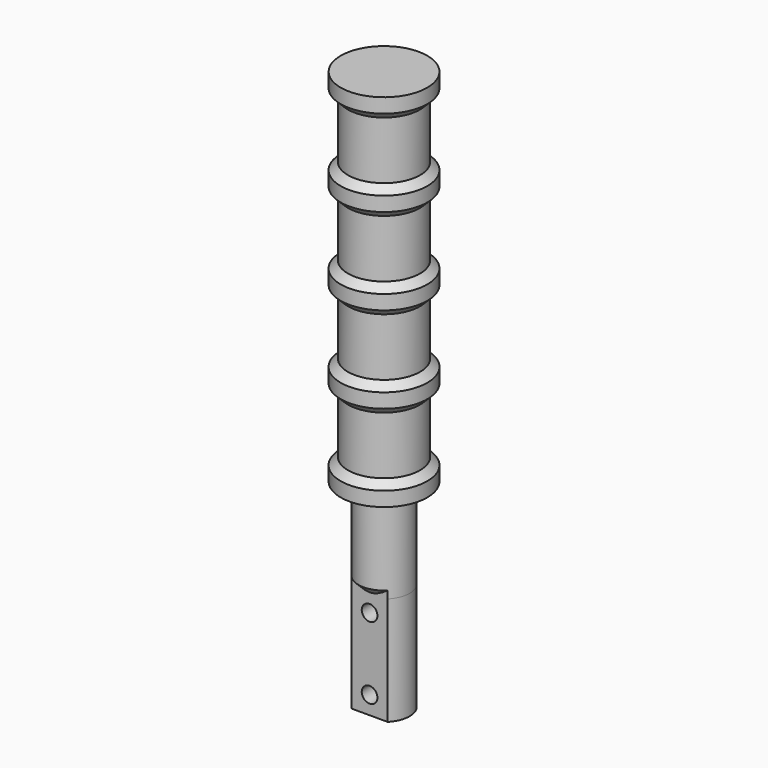
from build123d import *

# Parameters (mm, degrees)
F0_R         = 9.525
F1_DEPTH     = 152.4
F2_R         = 5.612663
F3_DEPTH     = 19.84375
F5_DEPTH     = 23.8125
F6_W         = 1.5875
F6_H         = 15.875
F6_W_2       = 9.525
F6_H_2       = 73.025
F8_R         = 1.7272
F9_DEPTH     = 7.937505
F10_T4_ANGLE = 176.348425
F10_T9_ANGLE = 176.348425
F11_SIZE     = 1.58749


# Not quite as in the source:
# - a fillet or chamfer that OpenCascade refuses, or shapes differently, is made with other operations: its cross-section is extruded or revolved along the edge and cut away or added
# - a fillet or chamfer is up to 0.001 mm smaller than in the source, because OpenCascade refuses the exact size


with BuildPart() as f1:
    # F0 (on Top) → F1 (new body)
    with BuildSketch(Plane.XY):
        Circle(F0_R)
    extrude(amount=F1_DEPTH)

    # F2 (on face) → F3 (join)
    with BuildSketch(Plane(origin=(0, 0, 0), x_dir=(1, 0, 0), z_dir=(0, 0, -1))):
        Circle(F2_R)
    extrude(amount=F3_DEPTH)

    # F4 (on face) → F5 (join)
    with BuildSketch(Plane(origin=(0, 0, -19.84375), x_dir=(1, 0, 0), z_dir=(0, 0, -1))):
        with BuildLine():
            ThreePointArc((3.968752, -3.968752), (5.612663, 0), (3.968752, 3.968752))
            Line((3.968752, 3.968752), (-3.968752, 3.968752))
            ThreePointArc((-3.968752, 3.968752), (-5.612663, 0), (-3.968752, -3.968752))
            Line((-3.968752, -3.968752), (3.968752, -3.968752))
        make_face()
    extrude(amount=F5_DEPTH)

    # F6 (on Front) → F7 (revolve, cut)
    with BuildSketch(Plane.XZ):
        with Locations((-8.73125, 11.1125)):
            Rectangle(F6_W, F6_H)
        with Locations((-8.73125, 30.1625)):
            Rectangle(F6_W, F6_H)
        with Locations((-8.73125, 49.2125)):
            Rectangle(F6_W, F6_H)
        with Locations((-8.73125, 68.2625)):
            Rectangle(F6_W, F6_H)
        with Locations((-4.7625, 115.8875)):
            Rectangle(F6_W_2, F6_H_2)
    revolve(axis=Axis((0, 0, 152.4), (0, 0, 1)), mode=Mode.SUBTRACT)

    # F8 (on face) → F9 (cut, through all)
    with BuildSketch(Plane.XZ.offset(3.968752)):
        with Locations((0, -39.6875)):
            Circle(F8_R)
        with Locations((0, -23.8125)):
            Circle(F8_R)
    extrude(amount=-F9_DEPTH, mode=Mode.SUBTRACT)

    # F10: chamfer of 1.643913 on 3 edges, made by hand


with BuildPart() as f10_tool2:
    # F10_s3 → F10_t4 (revolve)
    with BuildSketch(Plane(origin=(0, 0, 0), x_dir=(0, 0, 1), z_dir=(0.031861, 0.999492, 0))):
        Polygon((-18.199837, 5.612663), (-19.84375, 3.96875), (-19.84375, 5.612663), align=None)
    revolve(axis=Axis((0, 0, -19.84375), (0, 0, -1)), revolution_arc=F10_T4_ANGLE)

    split(bisect_by=Plane.XZ.offset(3.968752), keep=Keep.TOP)


with BuildPart() as f1_1:
    add(f1.part)

    # F10_t1: cut F10_tool2
    add(f10_tool2.part, mode=Mode.SUBTRACT)


with BuildPart() as f10_tool7:
    # F10_s8 → F10_t9 (revolve)
    with BuildSketch(Plane(origin=(0, 0, 0), x_dir=(0, 0, 1), z_dir=(-0.031861, -0.999492, 0))):
        Polygon((-18.199837, 5.612663), (-19.84375, 3.96875), (-19.84375, 5.612663), align=None)
    revolve(axis=Axis((0, 0, -19.84375), (0, 0, -1)), revolution_arc=F10_T9_ANGLE)

    split(bisect_by=Plane.XZ.offset(-3.968752), keep=Keep.BOTTOM)


with BuildPart() as f1_2:
    add(f1_1.part)

    # F10_t6: cut F10_tool7
    add(f10_tool7.part, mode=Mode.SUBTRACT)

    # F11 (size 1.5875 in the source; OpenCascade refuses exactly that, so slightly less here)
    f11_edges = [f1_2.edges().sort_by_distance(p)[0] for p in [
        (7.9375, 0, 3.175),
        (7.9375, 0, 19.05),
        (7.9375, 0, 38.1),
        (7.9375, 0, 57.15),
        (7.9375, 0, 76.2),
        (7.9375, 0, 60.325),
        (7.9375, 0, 41.275),
        (7.9375, 0, 22.225),
    ]]
    chamfer(f11_edges, length=F11_SIZE)


solid = f1_2.part
